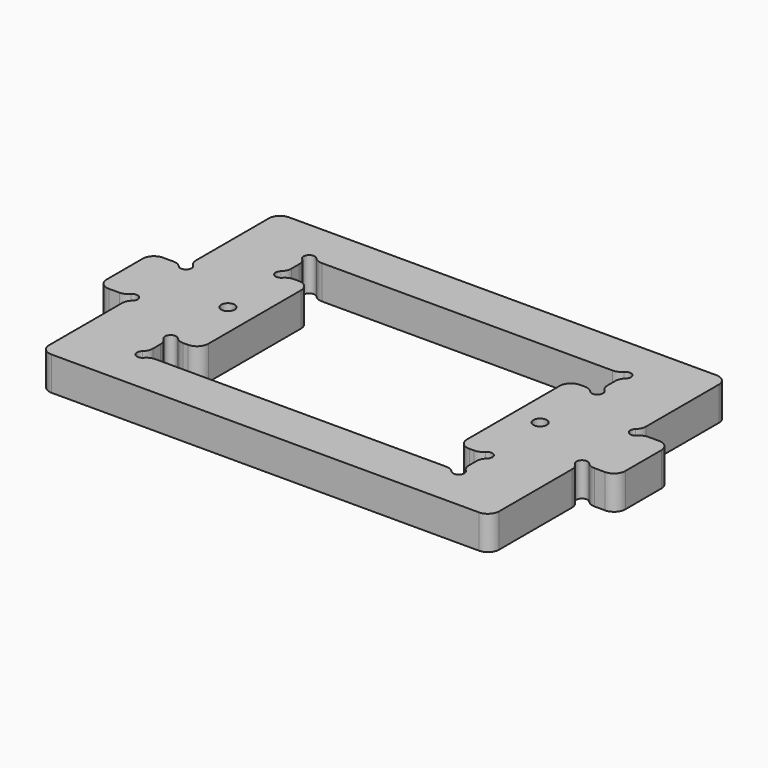
from build123d import *

# Parameters (mm, degrees)
F0_R     = 0.6
F1_DEPTH = 3
F2_W     = 3.05
F2_H     = 6
F3_DEPTH = 3
F5_D     = 1
F6_R     = 1


with BuildPart() as f1:
    # F0 (on Top) → F1 (new body)
    with BuildSketch(Plane.XY):
        Polygon((-20, 13.2), (-20, -13.2), (0, -13.2), (20, -13.2), (20, 13.2), align=None)
        with Locations((-13.875, 0)):
            Circle(F0_R, mode=Mode.SUBTRACT)
        Polygon((-14.05, 6.15), (-14.05, 9.25), (14.05, 9.25), (14.05, 6.15), (11.5, 6.15), (11.5, -6.15), (14.05, -6.15), (14.05, -9.25), (-14.05, -9.25), (-14.05, -6.15), (-11.5, -6.15), (-11.5, 6.15), align=None, mode=Mode.SUBTRACT)
        with Locations((13.875, 0)):
            Circle(F0_R, mode=Mode.SUBTRACT)
    extrude(amount=F1_DEPTH)

    # F2 (on face) → F3 (join, through all)
    with BuildSketch(Plane(origin=(0, 0, 0), x_dir=(1, 0, 0), z_dir=(0, 0, -1))):
        with Locations((-21.525, 0)):
            Rectangle(F2_W, F2_H)
        with Locations((21.525, 0)):
            Rectangle(F2_W, F2_H)
    extrude(amount=-F3_DEPTH)

    # F5 (through all)
    with Locations(Plane.XY.offset(3)):
        with Locations((-14.05, 9.25), (-14.05, 6.15), (-20, 3), (-20, -3), (-14.05, -6.15), (-14.05, -9.25), (14.05, -6.15), (14.05, -9.25), (20, -3), (20, 3), (14.05, 6.15), (14.05, 9.25)):
            Hole(F5_D / 2)

    # F6
    f6_edges = [f1.edges().sort_by_distance(p)[0] for p in [
        (-20, 13.2, 1.5),
        (-23.05, 3, 1.5),
        (-23.05, -3, 1.5),
        (-20, -13.2, 1.5),
        (-11.5, 6.15, 1.5),
        (11.5, -6.15, 1.5),
        (11.5, 6.15, 1.5),
        (23.05, 3, 1.5),
        (20, 13.2, 1.5),
        (23.05, -3, 1.5),
        (20, -13.2, 1.5),
        (-11.5, -6.15, 1.5),
        (-20, 3.5, 1.5),
        (20, 3.5, 1.5),
        (20.5, 3, 1.5),
        (20.5, -3, 1.5),
        (20, -3.5, 1.5),
        (-20, -3.5, 1.5),
        (-20.5, -3, 1.5),
        (-20.5, 3, 1.5),
        (-13.55, 6.15, 1.5),
        (-13.55, -6.15, 1.5),
        (-14.05, -6.65, 1.5),
        (-14.05, -8.75, 1.5),
        (-13.55, -9.25, 1.5),
        (13.55, -9.25, 1.5),
        (14.05, -8.75, 1.5),
        (14.05, -6.65, 1.5),
        (13.55, -6.15, 1.5),
        (13.55, 6.15, 1.5),
        (14.05, 6.65, 1.5),
        (14.05, 8.75, 1.5),
        (13.55, 9.25, 1.5),
        (-13.55, 9.25, 1.5),
        (-14.05, 8.75, 1.5),
        (-14.05, 6.65, 1.5),
    ]]
    fillet(f6_edges, radius=F6_R)


solid = f1.part
